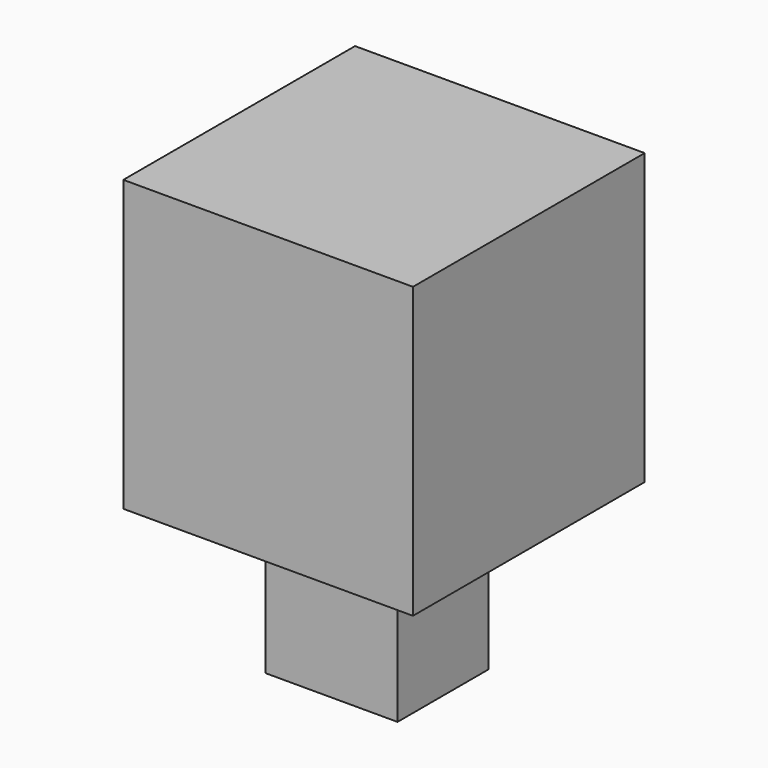
from build123d import *

# Parameters (mm, degrees)
F0_W     = 100
F0_H     = 100
F1_DEPTH = 100
F2_W     = 45.6354245543
F2_H     = 39.2044447362
F3_DEPTH = 154


# Not quite as in the source:
# - a feature names something its author has since deleted; it is built from what else it names


with BuildPart() as f1:
    # F0 (on Top) → F1 (new body)
    with BuildSketch(Plane.XY):
        with Locations((50, 50)):
            Rectangle(F0_W, F0_H)
    extrude(amount=F1_DEPTH)

    # F2 (on face) → F3 (join)
    with BuildSketch(Plane.XY.offset(100)):
        with Locations((47.8344149888, 49.6286619455)):
            Rectangle(F2_W, F2_H)
    extrude(amount=-F3_DEPTH)


solid = f1.part
